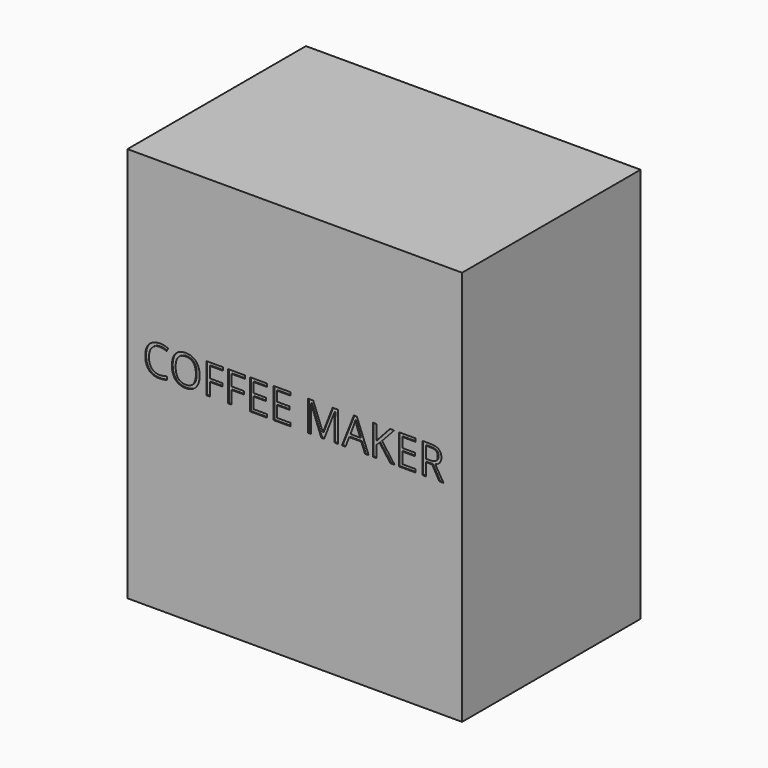
from build123d import *

# Parameters (mm, degrees)
F0_W         = 330
F0_H         = 220
F1_DEPTH     = 390
F2_TEXT_SIZE = 41.6666666667
F3_DEPTH     = 1


# Not quite as in the source:
# - Text() gives the source's letters only with a copy of the font that has no kerning and outlines rounded to 1/6400 em; it was checked with that copy


with BuildPart() as f1:
    # F0 (on Top) → F1 (new body)
    with BuildSketch(Plane.XY):
        Rectangle(F0_W, F0_H)
    extrude(amount=F1_DEPTH)

    # F2 (on face) → F3 (cut)
    with BuildSketch(Plane.XZ.offset(110)):
        with Locations((-150, 201.5409012696)):
            Text('COFFEE MAKER', F2_TEXT_SIZE, font='Open Sans', text_align=(TextAlign.LEFT, TextAlign.BOTTOM))
    extrude(amount=-F3_DEPTH, mode=Mode.SUBTRACT)


solid = f1.part
